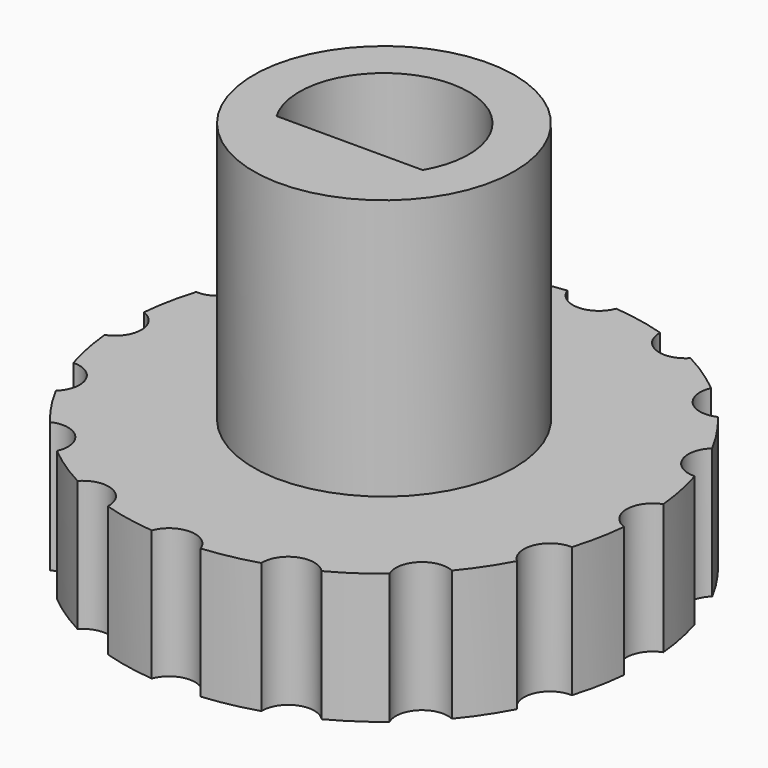
from build123d import *

# Parameters (mm, degrees)
F0_R            = 10
F1_DEPTH        = 5
F3_DEPTH        = 25
F3_COPIES_COUNT = 16
F5_R            = 5
F6_DEPTH        = 10


# Not quite as in the source:
# - a pattern or mirror of a feature is missing from the dataset's text; its kind, count and spacing are read off the source's solid


with BuildPart() as f1:
    # F0 (on Top) → F1 (new body)
    with BuildSketch(Plane.XY):
        Circle(F0_R)
    extrude(amount=F1_DEPTH)

    # F2 (on face) → F3 (cut)
    with BuildSketch(Plane.XY.offset(5)):
        with BuildLine():
            ThreePointArc((-0.9389056057, -9.9558252427), (0, -10), (0.9389056057, -9.9558252427))
            ThreePointArc((0.9389056057, -9.9558252427), (0, -9.3), (-0.9389056057, -9.9558252427))
        make_face()
    f3 = extrude(amount=-F3_DEPTH, mode=Mode.SUBTRACT)

    # F3_copies: F3 ×16 about axis
    f3_copies_axis = Axis((0, 0, 0), (0, 0, 1))
    for i in range(1, F3_COPIES_COUNT):
        add(f3.rotate(f3_copies_axis, i * 360 / F3_COPIES_COUNT), mode=Mode.SUBTRACT)

    # F5 (on face) → F6 (join)
    with BuildSketch(Plane.XY.offset(5)):
        Circle(F5_R)
        with BuildLine():
            ThreePointArc((-2.8, -1.65), (0, 3.25), (2.8, -1.65))
            Line((2.8, -1.65), (-2.8, -1.65))
        make_face(mode=Mode.SUBTRACT)
    extrude(amount=F6_DEPTH)


solid = f1.part
